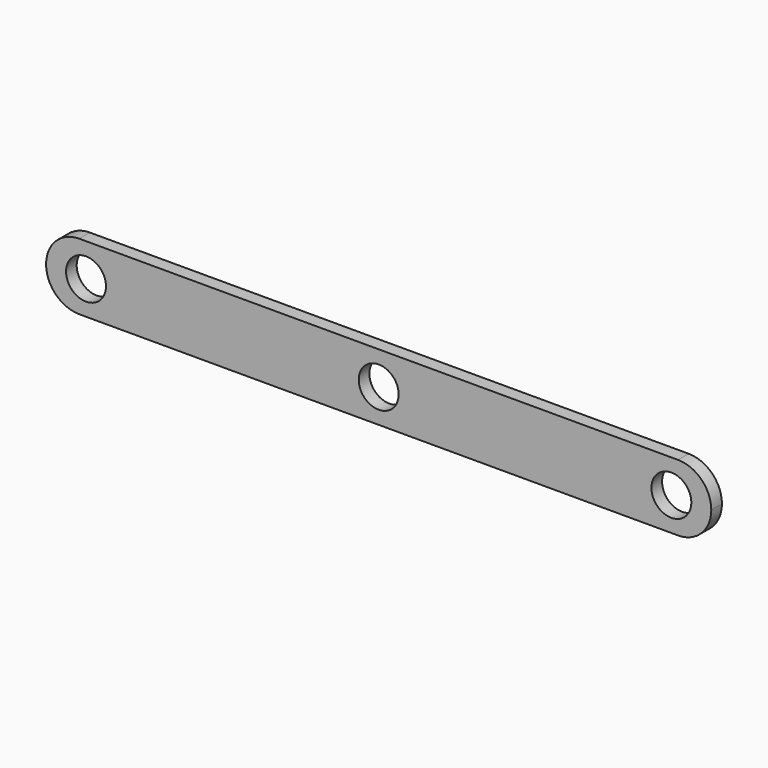
from build123d import *

# Parameters (mm, degrees)
F0_W     = 100
F0_H     = 10
F0_R     = 3
F1_DEPTH = 2
F2_R     = 4.99999


# Not quite as in the source:
# - a fillet or chamfer is up to 0.001 mm smaller than in the source, because OpenCascade refuses the exact size


with BuildPart() as f1:
    # F0 (on Front) → F1 (new body)
    with BuildSketch(Plane.XZ):
        Rectangle(F0_W, F0_H)
        with Locations((-44, 0)):
            Circle(F0_R, mode=Mode.SUBTRACT)
        Circle(F0_R, mode=Mode.SUBTRACT)
        with Locations((44, 0)):
            Circle(F0_R, mode=Mode.SUBTRACT)
    extrude(amount=F1_DEPTH)

    # F2 (radius 5 in the source; OpenCascade refuses exactly that, so slightly less here)
    f2_edges = [f1.edges().sort_by_distance(p)[0] for p in [
        (-50, -1, 5),
        (-50, -1, -5),
        (50, -1, 5),
        (50, -1, -5),
    ]]
    fillet(f2_edges, radius=F2_R)


solid = f1.part
